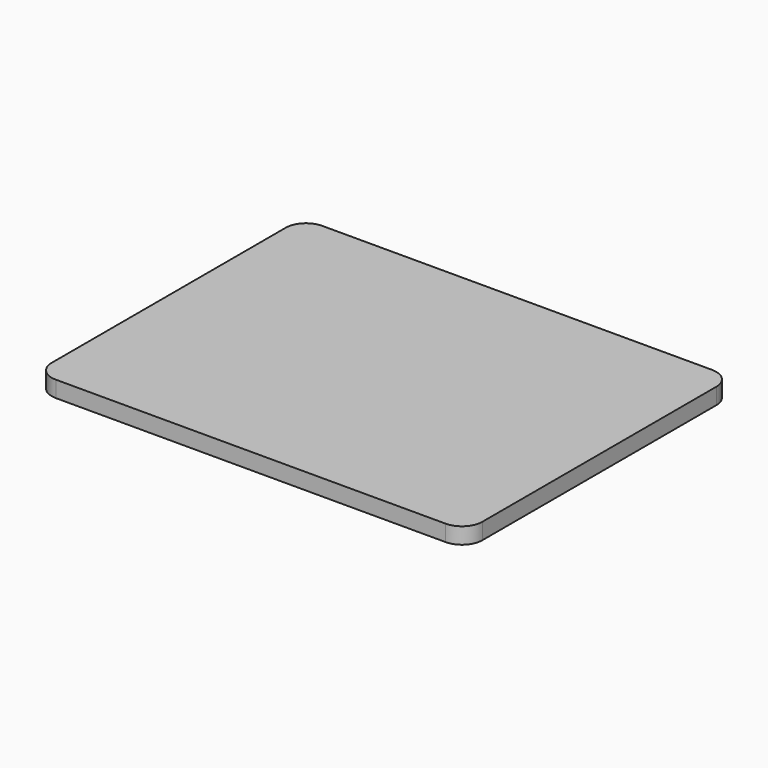
from build123d import *

# Parameters (mm, degrees)
F0_W     = 106
F0_H     = 82
F1_DEPTH = 4
F2_R     = 5


# Not quite as in the source:
# - a feature names something its author has since deleted; it is built from what else it names


with BuildPart() as f1:
    # F0 (on Top) → F1 (new body)
    with BuildSketch(Plane.XY):
        with Locations((0, -43.5)):
            Rectangle(F0_W, F0_H)
    extrude(amount=F1_DEPTH)

    # F2
    f2_edges = [f1.edges().sort_by_distance(p)[0] for p in [
        (53, -84.5, 2),
        (-53, -84.5, 2),
        (-53, -2.5, 2),
        (53, -2.5, 2),
    ]]
    fillet(f2_edges, radius=F2_R)


solid = f1.part
